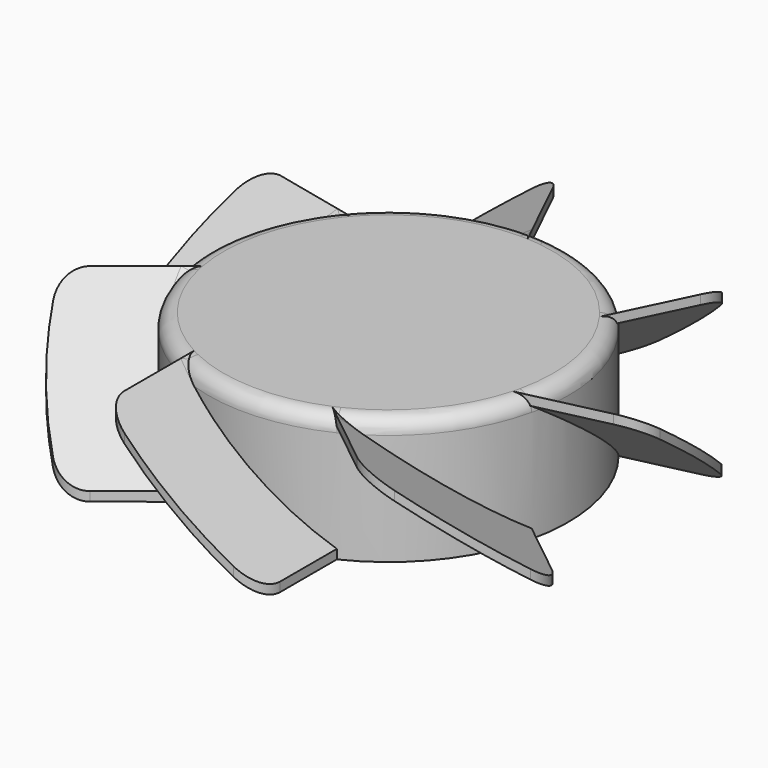
from build123d import *

# Parameters (mm, degrees)
F1_DEPTH       = 8.5
F3_DEPTH       = 10
F5_DEPTH       = 10
F7_DEPTH       = 10
F9_DEPTH       = 10
F11_DEPTH      = 10
F13_DEPTH      = 10
F15_DEPTH      = 10
F16_R          = 12.1
F17_DEPTH      = 8.5
F18_R          = 25
F18_R_2        = 18
F19_DEPTH      = 8.5
F20_R          = 2.5
F21_DEPTH      = 5
F22_T1_DEPTH   = 8.8499746994
F22_T3_DEPTH   = 8.8499746994
F23_T4_ANGLE   = 51.4285714286
F23_T9_ANGLE   = 51.4285714286
F23_T15_ANGLE  = 51.4285714286
F23_T21_ANGLE  = 51.4285714286
F23_T26_ANGLE  = 51.4285714286
F23_T32_ANGLE  = 51.4285714286
F23_T38_ANGLE  = 51.4285714286
F23_T43_ANGLE  = 51.4285714286
F23_T48_ANGLE  = 51.4285714286
F23_T53_ANGLE  = 51.4285714286
F23_T59_ANGLE  = 51.4285714286
F23_T65_ANGLE  = 51.4285714286
F23_T70_ANGLE  = 51.4285714286
F23_T75_ANGLE  = 51.4285714286
F23_T81_ANGLE  = 51.4285714286
F23_T87_ANGLE  = 51.4285714286
F23_T92_ANGLE  = 51.4285714286
F23_T97_ANGLE  = 51.4285714286
F23_T103_ANGLE = 51.4285714286
F23_T109_ANGLE = 51.4285714286
F23_T114_ANGLE = 51.4285714286
F23_T119_ANGLE = 51.4285714286
F23_T125_ANGLE = 51.4285714286
F23_T131_ANGLE = 51.4285714286
F23_T136_ANGLE = 51.4285714286
F23_T141_ANGLE = 51.4285714286
F23_T147_ANGLE = 51.4285714286
F23_T153_ANGLE = 51.4285714286


# Not quite as in the source:
# - a fillet or chamfer that OpenCascade refuses, or shapes differently, is made with other operations: its cross-section is extruded or revolved along the edge and cut away or added


with BuildPart() as f1:
    # F0 (on Top) → F1 (new body)
    with BuildSketch(Plane.XY):
        Polygon((9.4601609379, 7.5442266025), (0, 12.1), (-9.4601609379, 7.5442266025), (-11.7966277374, -2.6925033009), (-5.2499932433, -10.9017233016), (5.2499932433, -10.9017233016), (11.7966277374, -2.6925033009), align=None)
    extrude(amount=F1_DEPTH)

    # F2 (on face) → F3 (join)
    with BuildSketch(Plane(origin=(-10.6283943376, 2.4258616508, 0), x_dir=(-0.222520934, -0.9749279122, 0), z_dir=(-0.9749279122, 0.222520934, 0))):
        Polygon((5.2499932433, 0.6250002815), (-5.2499932433, 8.5), (-5.2499932433, 7.8749997185), (5.2499932433, 0), align=None)
    extrude(amount=F3_DEPTH)

    # F4 (on face) → F5 (join)
    with BuildSketch(Plane(origin=(-8.5233104904, -6.7971133012, 0), x_dir=(0.6234898019, -0.7818314825, 0), z_dir=(-0.7818314825, -0.6234898019, 0))):
        Polygon((5.2499932433, 0.6250002815), (-5.2499932433, 8.5), (-5.2499932433, 7.8749997185), (5.2499932433, 0), align=None)
    extrude(amount=F5_DEPTH)

    # F6 (on face) → F7 (join)
    with BuildSketch(Plane.XZ.offset(10.9017233016)):
        Polygon((5.2499932433, 0.6250002815), (-5.2499932433, 8.5), (-5.2499932433, 7.8749997185), (5.2499932433, 0), align=None)
    extrude(amount=F7_DEPTH)

    # F8 (on face) → F9 (join)
    with BuildSketch(Plane(origin=(8.5233104904, -6.7971133012, 0), x_dir=(0.6234898019, 0.7818314825, 0), z_dir=(0.7818314825, -0.6234898019, 0))):
        Polygon((5.2499932433, 0.6250002815), (-5.2499932433, 8.5), (-5.2499932433, 7.8749997185), (5.2499932433, 0), align=None)
    extrude(amount=F9_DEPTH)

    # F10 (on face) → F11 (join)
    with BuildSketch(Plane(origin=(10.6283943376, 2.4258616508, 0), x_dir=(-0.222520934, 0.9749279122, 0), z_dir=(0.9749279122, 0.222520934, 0))):
        Polygon((5.2499932433, 0.6250002815), (-5.2499932433, 8.5), (-5.2499932433, 7.8749997185), (5.2499932433, 0), align=None)
    extrude(amount=F11_DEPTH)

    # F12 (on face) → F13 (join)
    with BuildSketch(Plane(origin=(4.7300804689, 9.8221133012, 0), x_dir=(-0.9009688679, 0.4338837391, 0), z_dir=(0.4338837391, 0.9009688679, 0))):
        Polygon((5.2499932433, 0.6250002815), (-5.2499932433, 8.5), (-5.2499932433, 7.8749997185), (5.2499932433, 0), align=None)
    extrude(amount=F13_DEPTH)

    # F14 (on face) → F15 (join)
    with BuildSketch(Plane(origin=(-4.7300804689, 9.8221133012, 0), x_dir=(-0.9009688679, -0.4338837391, 0), z_dir=(-0.4338837391, 0.9009688679, 0))):
        Polygon((5.2499932433, 0.6250002815), (-5.2499932433, 8.5), (-5.2499932433, 7.8749997185), (5.2499932433, 0), align=None)
    extrude(amount=F15_DEPTH)

    # F16 (on Top) → F17 (join)
    with BuildSketch(Plane.XY):
        Circle(F16_R)
    extrude(amount=F17_DEPTH)

    # F18 (on face) → F19 (cut, through all)
    with BuildSketch(Plane.XY.offset(8.5)):
        Circle(F18_R)
        Circle(F18_R_2, mode=Mode.SUBTRACT)
    extrude(amount=-F19_DEPTH, mode=Mode.SUBTRACT)

    # F20 (on face) → F21 (cut)
    with BuildSketch(Plane(origin=(0, 0, 0), x_dir=(1, 0, 0), z_dir=(0, 0, -1))):
        Circle(F20_R)
    extrude(amount=-F21_DEPTH, mode=Mode.SUBTRACT)

    # F22: fillet of radius 2 on 14 edges, made by hand

    # F22_s2 → F22_t1 (cut)
    with BuildSketch(Plane.XY.offset(3.7625125095)):
        with BuildLine():
            ThreePointArc((-5.2499932433, -15.6664464356), (-4.8012021768, -16.9288848874), (-3.6562423987, -17.62475224))
            ThreePointArc((-3.6562423987, -17.62475224), (-4.4577741005, -17.4392732093), (-5.2499932433, -17.2173624852))
            Line((-5.2499932433, -17.2173624852), (-5.2499932433, -15.6664464356))
        make_face()
        with BuildLine():
            ThreePointArc((8.9752037947, -13.8724795843), (10.2420345741, -14.3087180997), (11.4999563232, -13.8474186968))
            ThreePointArc((11.4999563232, -13.8474186968), (10.8551961357, -14.3584371313), (10.1877587889, -14.8394599248))
            Line((10.1877587889, -14.8394599248), (8.9752037947, -13.8724795843))
        make_face()
        with BuildLine():
            ThreePointArc((16.4418893145, -1.6322526591), (17.5728103913, -0.9137947383), (17.9964533774, 0.357303561))
            ThreePointArc((17.9964533774, 0.357303561), (17.9939822761, -0.4654050347), (17.9539206607, -1.2871413712))
            Line((17.9539206607, -1.2871413712), (16.4418893145, -1.6322526591))
        make_face()
        with BuildLine():
            ThreePointArc((11.5274968271, 11.8370938103), (11.6709015639, 13.1692346991), (10.9412539777, 14.2929689497))
            ThreePointArc((10.9412539777, 14.2929689497), (11.5829327522, 13.7780865456), (12.2004140817, 13.2344208878))
            Line((12.2004140817, 13.2344208878), (11.5274968271, 11.8370938103))
        make_face()
        with BuildLine():
            ThreePointArc((-2.0673358892, 16.3928672079), (-3.0194341842, 17.3355618046), (-4.3529328281, 17.4657371958))
            ThreePointArc((-4.3529328281, 17.4657371958), (-3.5503013829, 17.6463979353), (-2.7402531439, 17.7901942853))
            Line((-2.7402531439, 17.7901942853), (-2.0673358892, 16.3928672079))
        make_face()
        with BuildLine():
            ThreePointArc((-14.105422515, 8.6044772443), (-15.4360744063, 8.4478572902), (-16.3692724307, 7.4864490974))
            ThreePointArc((-16.3692724307, 7.4864490974), (-16.0100861637, 8.2266117588), (-15.6174538612, 8.9495885321))
            Line((-15.6174538612, 8.9495885321), (-14.105422515, 8.6044772443))
        make_face()
        with BuildLine():
            ThreePointArc((-15.5218382888, -5.6632595836), (-16.2290357619, -6.8012560686), (-16.0592160207, -8.1302878671))
            ThreePointArc((-16.0592160207, -8.1302878671), (-16.413949517, -7.3879808643), (-16.734393283, -6.630239924))
            Line((-16.734393283, -6.630239924), (-15.5218382888, -5.6632595836))
        make_face()
    extrude(amount=F22_T1_DEPTH, mode=Mode.SUBTRACT)

    # F22_s4 → F22_t3 (cut)
    with BuildSketch(Plane.XY.offset(-4.1124872089)):
        with BuildLine():
            ThreePointArc((5.2499932433, -15.6664464356), (4.8012021768, -16.9288848874), (3.6562423987, -17.62475224))
            ThreePointArc((3.6562423987, -17.62475224), (4.4577741005, -17.4392732093), (5.2499932433, -17.2173624852))
            Line((5.2499932433, -17.2173624852), (5.2499932433, -15.6664464356))
        make_face()
        with BuildLine():
            ThreePointArc((15.5218382888, -5.6632595836), (16.2290357619, -6.8012560686), (16.0592160207, -8.1302878671))
            ThreePointArc((16.0592160207, -8.1302878671), (16.413949517, -7.3879808643), (16.734393283, -6.630239924))
            Line((16.734393283, -6.630239924), (15.5218382888, -5.6632595836))
        make_face()
        with BuildLine():
            ThreePointArc((14.105422515, 8.6044772443), (15.4360744063, 8.4478572902), (16.3692724307, 7.4864490974))
            ThreePointArc((16.3692724307, 7.4864490974), (16.0100861637, 8.2266117588), (15.6174538612, 8.9495885321))
            Line((15.6174538612, 8.9495885321), (14.105422515, 8.6044772443))
        make_face()
        with BuildLine():
            ThreePointArc((2.0673358892, 16.3928672079), (3.0194341842, 17.3355618046), (4.3529328281, 17.4657371958))
            ThreePointArc((4.3529328281, 17.4657371958), (3.5503013829, 17.6463979353), (2.7402531439, 17.7901942853))
            Line((2.7402531439, 17.7901942853), (2.0673358892, 16.3928672079))
        make_face()
        with BuildLine():
            ThreePointArc((-11.5274968271, 11.8370938103), (-11.6709015639, 13.1692346991), (-10.9412539777, 14.2929689497))
            ThreePointArc((-10.9412539777, 14.2929689497), (-11.5829327522, 13.7780865456), (-12.2004140817, 13.2344208878))
            Line((-12.2004140817, 13.2344208878), (-11.5274968271, 11.8370938103))
        make_face()
        with BuildLine():
            ThreePointArc((-16.4418893145, -1.6322526591), (-17.5728103913, -0.9137947383), (-17.9964533774, 0.357303561))
            ThreePointArc((-17.9964533774, 0.357303561), (-17.9939822761, -0.4654050347), (-17.9539206607, -1.2871413712))
            Line((-17.9539206607, -1.2871413712), (-16.4418893145, -1.6322526591))
        make_face()
        with BuildLine():
            ThreePointArc((-8.9752037947, -13.8724795843), (-10.2420345741, -14.3087180997), (-11.4999563232, -13.8474186968))
            ThreePointArc((-11.4999563232, -13.8474186968), (-10.8551961357, -14.3584371313), (-10.1877587889, -14.8394599248))
            Line((-10.1877587889, -14.8394599248), (-8.9752037947, -13.8724795843))
        make_face()
    extrude(amount=F22_T3_DEPTH, mode=Mode.SUBTRACT)

    # F23: fillet of radius 1 on 7 edges, made by hand


with BuildPart() as f23_tool2:
    # F23_s3 → F23_t4 (revolve)
    with BuildSketch(Plane(origin=(0, 0, 0), x_dir=(0, 0, 1), z_dir=(-0.9009688679, -0.4338837391, 0))):
        with BuildLine():
            ThreePointArc((7.5, -12.1), (8.2071067812, -11.8071067812), (8.5, -11.1))
            Line((8.5, -11.1), (8.5, -12.1))
            Line((8.5, -12.1), (7.5, -12.1))
        make_face()
    revolve(axis=Axis((0, 0, 8.5), (0, 0, 1)), revolution_arc=F23_T4_ANGLE)

    split(bisect_by=Plane(origin=(1.1783960962, 1.4776619667, 2.5199976397), x_dir=(0.7818314825, -0.6234898019, 0), z_dir=(-0.3740941807, -0.4690992651, -0.7999996396)), keep=Keep.TOP)


with BuildPart() as f1_1:
    add(f1.part)

    # F23_t1: cut F23_tool2
    add(f23_tool2.part, mode=Mode.SUBTRACT)


with BuildPart() as f23_tool7:
    # F23_s8 → F23_t9 (revolve)
    with BuildSketch(Plane(origin=(0, 0, 0), x_dir=(0, 0, 1), z_dir=(-0.9009688679, -0.4338837391, 0))):
        with BuildLine():
            ThreePointArc((7.5, -12.1), (8.2071067812, -11.8071067812), (8.5, -11.1))
            Line((8.5, -11.1), (8.5, -12.1))
            Line((8.5, -12.1), (7.5, -12.1))
        make_face()
    revolve(axis=Axis((0, 0, 8.5), (0, 0, 1)), revolution_arc=F23_T9_ANGLE)

    split(bisect_by=Plane(origin=(1.3654431866, 1.7122115993, 2.9199974595), x_dir=(-0.7818314825, 0.6234898019, 0), z_dir=(0.3740941807, 0.4690992651, 0.7999996396)), keep=Keep.TOP)

    split(bisect_by=Plane(origin=(1.1682333998, -5.1183649517, 0), x_dir=(0, 0, 1), z_dir=(0.222520934, -0.9749279122, 0)), keep=Keep.TOP)


with BuildPart() as f1_2:
    add(f1_1.part)

    # F23_t6: cut F23_tool7
    add(f23_tool7.part, mode=Mode.SUBTRACT)


with BuildPart() as f23_tool13:
    # F23_s14 → F23_t15 (revolve)
    with BuildSketch(Plane(origin=(0, 0, 0), x_dir=(0, 0, 1), z_dir=(-0.9009688679, -0.4338837391, 0))):
        with BuildLine():
            ThreePointArc((7.5, -12.1), (8.2071067812, -11.8071067812), (8.5, -11.1))
            Line((8.5, -11.1), (8.5, -12.1))
            Line((8.5, -12.1), (7.5, -12.1))
        make_face()
    revolve(axis=Axis((0, 0, 8.5), (0, 0, 1)), revolution_arc=F23_T15_ANGLE)

    split(bisect_by=Plane(origin=(-0.4205646975, 1.8426143337, 2.5199976397), x_dir=(0.9749279122, 0.222520934, 0), z_dir=(0.1335126673, -0.5849572157, -0.7999996396)), keep=Keep.TOP)

    split(bisect_by=Plane(origin=(1.1682333998, -5.1183649517, 0), x_dir=(0, 0, 1), z_dir=(-0.222520934, 0.9749279122, 0)), keep=Keep.TOP)


with BuildPart() as f1_3:
    add(f1_2.part)

    # F23_t12: cut F23_tool13
    add(f23_tool13.part, mode=Mode.SUBTRACT)


with BuildPart() as f23_tool19:
    # F23_s20 → F23_t21 (revolve)
    with BuildSketch(Plane(origin=(0, 0, 0), x_dir=(0, 0, 1), z_dir=(-0.9009688679, -0.4338837391, 0))):
        with BuildLine():
            ThreePointArc((7.5, -12.1), (8.2071067812, -11.8071067812), (8.5, -11.1))
            Line((8.5, -11.1), (8.5, -12.1))
            Line((8.5, -12.1), (7.5, -12.1))
        make_face()
    revolve(axis=Axis((0, 0, 8.5), (0, 0, 1)), revolution_arc=F23_T21_ANGLE)

    split(bisect_by=Plane(origin=(-0.4873210311, 2.1350929416, 2.9199974595), x_dir=(-0.9749279122, -0.222520934, 0), z_dir=(-0.1335126673, 0.5849572157, 0.7999996396)), keep=Keep.TOP)


with BuildPart() as f1_4:
    add(f1_3.part)

    # F23_t18: cut F23_tool19
    add(f23_tool19.part, mode=Mode.SUBTRACT)


with BuildPart() as f23_tool24:
    # F23_s25 → F23_t26 (revolve)
    with BuildSketch(Plane(origin=(0, 0, 0), x_dir=(0, 0, 1), z_dir=(-0.6234898019, 0.7818314825, 0))):
        with BuildLine():
            ThreePointArc((7.5, 12.1), (8.2071067812, 11.8071067812), (8.5, 11.1))
            Line((8.5, 11.1), (8.5, 12.1))
            Line((8.5, 12.1), (7.5, 12.1))
        make_face()
    revolve(axis=Axis((0, 0, 8.5), (0, 0, -1)), revolution_arc=F23_T26_ANGLE)

    split(bisect_by=Plane(origin=(-0.4873210311, 2.1350929416, 2.9199974595), x_dir=(-0.9749279122, -0.222520934, 0), z_dir=(-0.1335126673, 0.5849572157, 0.7999996396)), keep=Keep.TOP)

    split(bisect_by=Plane(origin=(-1.702831696, 0.8200405249, 2.5199976397), x_dir=(0.4338837391, 0.9009688679, 0), z_dir=(0.5405817536, -0.2603304519, -0.7999996396)), keep=Keep.TOP)


with BuildPart() as f1_5:
    add(f1_4.part)

    # F23_t23: cut F23_tool24
    add(f23_tool24.part, mode=Mode.SUBTRACT)


with BuildPart() as f23_tool30:
    # F23_s31 → F23_t32 (revolve)
    with BuildSketch(Plane(origin=(0, 0, 0), x_dir=(0, 0, 1), z_dir=(-0.6234898019, 0.7818314825, 0))):
        with BuildLine():
            ThreePointArc((7.5, 12.1), (8.2071067812, 11.8071067812), (8.5, 11.1))
            Line((8.5, 11.1), (8.5, 12.1))
            Line((8.5, 12.1), (7.5, 12.1))
        make_face()
    revolve(axis=Axis((0, 0, 8.5), (0, 0, -1)), revolution_arc=F23_T32_ANGLE)

    split(bisect_by=Plane(origin=(4.7300804689, -2.2778866988, 0), x_dir=(0, 0, 1), z_dir=(0.9009688679, -0.4338837391, 0)), keep=Keep.TOP)

    split(bisect_by=Plane(origin=(-1.702831696, 0.8200405249, 2.5199976397), x_dir=(-0.4338837391, -0.9009688679, 0), z_dir=(-0.5405817536, 0.2603304519, 0.7999996396)), keep=Keep.TOP)


with BuildPart() as f1_6:
    add(f1_5.part)

    # F23_t29: cut F23_tool30
    add(f23_tool30.part, mode=Mode.SUBTRACT)


with BuildPart() as f23_tool36:
    # F23_s37 → F23_t38 (revolve)
    with BuildSketch(Plane(origin=(0, 0, 0), x_dir=(0, 0, 1), z_dir=(-0.6234898019, 0.7818314825, 0))):
        with BuildLine():
            ThreePointArc((7.5, 12.1), (8.2071067812, 11.8071067812), (8.5, 11.1))
            Line((8.5, 11.1), (8.5, 12.1))
            Line((8.5, 12.1), (7.5, 12.1))
        make_face()
    revolve(axis=Axis((0, 0, 8.5), (0, 0, -1)), revolution_arc=F23_T38_ANGLE)

    split(bisect_by=Plane(origin=(-0.4205646975, 1.8426143337, 2.5199976397), x_dir=(0.9749279122, 0.222520934, 0), z_dir=(0.1335126673, -0.5849572157, -0.7999996396)), keep=Keep.TOP)


with BuildPart() as f1_7:
    add(f1_6.part)

    # F23_t35: cut F23_tool36
    add(f23_tool36.part, mode=Mode.SUBTRACT)


with BuildPart() as f23_tool41:
    # F23_s42 → F23_t43 (revolve)
    with BuildSketch(Plane(origin=(0, 0, 0), x_dir=(0, 0, 1), z_dir=(-0.6234898019, 0.7818314825, 0))):
        with BuildLine():
            ThreePointArc((7.5, 12.1), (8.2071067812, 11.8071067812), (8.5, 11.1))
            Line((8.5, 11.1), (8.5, 12.1))
            Line((8.5, 12.1), (7.5, 12.1))
        make_face()
    revolve(axis=Axis((0, 0, 8.5), (0, 0, -1)), revolution_arc=F23_T43_ANGLE)

    split(bisect_by=Plane(origin=(-1.9731225729, 0.9502057509, 2.9199974595), x_dir=(-0.4338837391, -0.9009688679, 0), z_dir=(-0.5405817536, 0.2603304519, 0.7999996396)), keep=Keep.TOP)


with BuildPart() as f1_8:
    add(f1_7.part)

    # F23_t40: cut F23_tool41
    add(f23_tool41.part, mode=Mode.SUBTRACT)


with BuildPart() as f23_tool46:
    # F23_s47 → F23_t48 (revolve)
    with BuildSketch(Plane(origin=(0, 0, 0), x_dir=(0, 0, 1), z_dir=(0.6234898019, -0.7818314825, 0))):
        with BuildLine():
            ThreePointArc((7.5, -12.1), (8.2071067812, -11.8071067812), (8.5, -11.1))
            Line((8.5, -11.1), (8.5, -12.1))
            Line((8.5, -12.1), (7.5, -12.1))
        make_face()
    revolve(axis=Axis((0, 0, 8.5), (0, 0, 1)), revolution_arc=F23_T48_ANGLE)

    split(bisect_by=Plane(origin=(-1.702831696, 0.8200405249, 2.5199976397), x_dir=(0.4338837391, 0.9009688679, 0), z_dir=(0.5405817536, -0.2603304519, -0.7999996396)), keep=Keep.TOP)


with BuildPart() as f1_9:
    add(f1_8.part)

    # F23_t45: cut F23_tool46
    add(f23_tool46.part, mode=Mode.SUBTRACT)


with BuildPart() as f23_tool51:
    # F23_s52 → F23_t53 (revolve)
    with BuildSketch(Plane(origin=(0, 0, 0), x_dir=(0, 0, 1), z_dir=(0.6234898019, -0.7818314825, 0))):
        with BuildLine():
            ThreePointArc((7.5, -12.1), (8.2071067812, -11.8071067812), (8.5, -11.1))
            Line((8.5, -11.1), (8.5, -12.1))
            Line((8.5, -12.1), (7.5, -12.1))
        make_face()
    revolve(axis=Axis((0, 0, 8.5), (0, 0, 1)), revolution_arc=F23_T53_ANGLE)

    split(bisect_by=Plane(origin=(-1.9731225729, 0.9502057509, 2.9199974595), x_dir=(-0.4338837391, -0.9009688679, 0), z_dir=(-0.5405817536, 0.2603304519, 0.7999996396)), keep=Keep.TOP)

    split(bisect_by=Plane(origin=(-1.702831696, -0.8200405249, 2.5199976397), x_dir=(-0.4338837391, 0.9009688679, 0), z_dir=(0.5405817536, 0.2603304519, -0.7999996396)), keep=Keep.TOP)


with BuildPart() as f1_10:
    add(f1_9.part)

    # F23_t50: cut F23_tool51
    add(f23_tool51.part, mode=Mode.SUBTRACT)


with BuildPart() as f23_tool57:
    # F23_s58 → F23_t59 (revolve)
    with BuildSketch(Plane(origin=(0, 0, 0), x_dir=(0, 0, 1), z_dir=(0.6234898019, -0.7818314825, 0))):
        with BuildLine():
            ThreePointArc((7.5, -12.1), (8.2071067812, -11.8071067812), (8.5, -11.1))
            Line((8.5, -11.1), (8.5, -12.1))
            Line((8.5, -12.1), (7.5, -12.1))
        make_face()
    revolve(axis=Axis((0, 0, 8.5), (0, 0, 1)), revolution_arc=F23_T59_ANGLE)

    split(bisect_by=Plane(origin=(4.7300804689, 2.2778866988, 0), x_dir=(0, 0, 1), z_dir=(0.9009688679, 0.4338837391, 0)), keep=Keep.TOP)

    split(bisect_by=Plane(origin=(-1.702831696, -0.8200405249, 2.5199976397), x_dir=(0.4338837391, -0.9009688679, 0), z_dir=(-0.5405817536, -0.2603304519, 0.7999996396)), keep=Keep.TOP)


with BuildPart() as f1_11:
    add(f1_10.part)

    # F23_t56: cut F23_tool57
    add(f23_tool57.part, mode=Mode.SUBTRACT)


with BuildPart() as f23_tool63:
    # F23_s64 → F23_t65 (revolve)
    with BuildSketch(Plane(origin=(0, 0, 0), x_dir=(0, 0, 1), z_dir=(0.6234898019, -0.7818314825, 0))):
        with BuildLine():
            ThreePointArc((7.5, -12.1), (8.2071067812, -11.8071067812), (8.5, -11.1))
            Line((8.5, -11.1), (8.5, -12.1))
            Line((8.5, -12.1), (7.5, -12.1))
        make_face()
    revolve(axis=Axis((0, 0, 8.5), (0, 0, 1)), revolution_arc=F23_T65_ANGLE)

    split(bisect_by=Plane(origin=(-1.9731225729, -0.9502057509, 2.9199974595), x_dir=(0.4338837391, -0.9009688679, 0), z_dir=(-0.5405817536, -0.2603304519, 0.7999996396)), keep=Keep.TOP)


with BuildPart() as f1_12:
    add(f1_11.part)

    # F23_t62: cut F23_tool63
    add(f23_tool63.part, mode=Mode.SUBTRACT)


with BuildPart() as f23_tool68:
    # F23_s69 → F23_t70 (revolve)
    with BuildSketch(Plane.YZ):
        with BuildLine():
            ThreePointArc((12.1, 7.5), (11.8071067812, 8.2071067812), (11.1, 8.5))
            Line((11.1, 8.5), (12.1, 8.5))
            Line((12.1, 8.5), (12.1, 7.5))
        make_face()
    revolve(axis=Axis((0, 0, 8.5), (0, 0, 1)), revolution_arc=F23_T70_ANGLE)

    split(bisect_by=Plane(origin=(-1.702831696, -0.8200405249, 2.5199976397), x_dir=(-0.4338837391, 0.9009688679, 0), z_dir=(0.5405817536, 0.2603304519, -0.7999996396)), keep=Keep.TOP)


with BuildPart() as f1_13:
    add(f1_12.part)

    # F23_t67: cut F23_tool68
    add(f23_tool68.part, mode=Mode.SUBTRACT)


with BuildPart() as f23_tool73:
    # F23_s74 → F23_t75 (revolve)
    with BuildSketch(Plane.YZ):
        with BuildLine():
            ThreePointArc((12.1, 7.5), (11.8071067812, 8.2071067812), (11.1, 8.5))
            Line((11.1, 8.5), (12.1, 8.5))
            Line((12.1, 8.5), (12.1, 7.5))
        make_face()
    revolve(axis=Axis((0, 0, 8.5), (0, 0, 1)), revolution_arc=F23_T75_ANGLE)

    split(bisect_by=Plane(origin=(-1.9731225729, -0.9502057509, 2.9199974595), x_dir=(0.4338837391, -0.9009688679, 0), z_dir=(-0.5405817536, -0.2603304519, 0.7999996396)), keep=Keep.TOP)

    split(bisect_by=Plane(origin=(-0.4205646975, -1.8426143337, 2.5199976397), x_dir=(-0.9749279122, 0.222520934, 0), z_dir=(0.1335126673, 0.5849572157, -0.7999996396)), keep=Keep.TOP)


with BuildPart() as f1_14:
    add(f1_13.part)

    # F23_t72: cut F23_tool73
    add(f23_tool73.part, mode=Mode.SUBTRACT)


with BuildPart() as f23_tool79:
    # F23_s80 → F23_t81 (revolve)
    with BuildSketch(Plane.YZ):
        with BuildLine():
            ThreePointArc((12.1, 7.5), (11.8071067812, 8.2071067812), (11.1, 8.5))
            Line((11.1, 8.5), (12.1, 8.5))
            Line((12.1, 8.5), (12.1, 7.5))
        make_face()
    revolve(axis=Axis((0, 0, 8.5), (0, 0, 1)), revolution_arc=F23_T81_ANGLE)

    split(bisect_by=Plane(origin=(1.1682333998, 5.1183649517, 0), x_dir=(0, 0, 1), z_dir=(0.222520934, 0.9749279122, 0)), keep=Keep.TOP)

    split(bisect_by=Plane(origin=(-0.4205646975, -1.8426143337, 2.5199976397), x_dir=(0.9749279122, -0.222520934, 0), z_dir=(-0.1335126673, -0.5849572157, 0.7999996396)), keep=Keep.TOP)


with BuildPart() as f1_15:
    add(f1_14.part)

    # F23_t78: cut F23_tool79
    add(f23_tool79.part, mode=Mode.SUBTRACT)


with BuildPart() as f23_tool85:
    # F23_s86 → F23_t87 (revolve)
    with BuildSketch(Plane.YZ):
        with BuildLine():
            ThreePointArc((12.1, 7.5), (11.8071067812, 8.2071067812), (11.1, 8.5))
            Line((11.1, 8.5), (12.1, 8.5))
            Line((12.1, 8.5), (12.1, 7.5))
        make_face()
    revolve(axis=Axis((0, 0, 8.5), (0, 0, 1)), revolution_arc=F23_T87_ANGLE)

    split(bisect_by=Plane(origin=(-0.4873210311, -2.1350929416, 2.9199974595), x_dir=(0.9749279122, -0.222520934, 0), z_dir=(-0.1335126673, -0.5849572157, 0.7999996396)), keep=Keep.TOP)


with BuildPart() as f1_16:
    add(f1_15.part)

    # F23_t84: cut F23_tool85
    add(f23_tool85.part, mode=Mode.SUBTRACT)


with BuildPart() as f23_tool90:
    # F23_s91 → F23_t92 (revolve)
    with BuildSketch(Plane(origin=(0, 0, 0), x_dir=(0, 0, 1), z_dir=(0.6234898019, 0.7818314825, 0))):
        with BuildLine():
            ThreePointArc((7.5, -12.1), (8.2071067812, -11.8071067812), (8.5, -11.1))
            Line((8.5, -11.1), (8.5, -12.1))
            Line((8.5, -12.1), (7.5, -12.1))
        make_face()
    revolve(axis=Axis((0, 0, 8.5), (0, 0, 1)), revolution_arc=F23_T92_ANGLE)

    split(bisect_by=Plane(origin=(-0.4205646975, -1.8426143337, 2.5199976397), x_dir=(-0.9749279122, 0.222520934, 0), z_dir=(0.1335126673, 0.5849572157, -0.7999996396)), keep=Keep.TOP)


with BuildPart() as f1_17:
    add(f1_16.part)

    # F23_t89: cut F23_tool90
    add(f23_tool90.part, mode=Mode.SUBTRACT)


with BuildPart() as f23_tool95:
    # F23_s96 → F23_t97 (revolve)
    with BuildSketch(Plane(origin=(0, 0, 0), x_dir=(0, 0, 1), z_dir=(0.6234898019, 0.7818314825, 0))):
        with BuildLine():
            ThreePointArc((7.5, -12.1), (8.2071067812, -11.8071067812), (8.5, -11.1))
            Line((8.5, -11.1), (8.5, -12.1))
            Line((8.5, -12.1), (7.5, -12.1))
        make_face()
    revolve(axis=Axis((0, 0, 8.5), (0, 0, 1)), revolution_arc=F23_T97_ANGLE)

    split(bisect_by=Plane(origin=(-0.4873210311, -2.1350929416, 2.9199974595), x_dir=(0.9749279122, -0.222520934, 0), z_dir=(-0.1335126673, -0.5849572157, 0.7999996396)), keep=Keep.TOP)

    split(bisect_by=Plane(origin=(-3.273317247, 4.1046100004, 0), x_dir=(0, 0, 1), z_dir=(-0.6234898019, 0.7818314825, 0)), keep=Keep.TOP)


with BuildPart() as f1_18:
    add(f1_17.part)

    # F23_t94: cut F23_tool95
    add(f23_tool95.part, mode=Mode.SUBTRACT)


with BuildPart() as f23_tool101:
    # F23_s102 → F23_t103 (revolve)
    with BuildSketch(Plane(origin=(0, 0, 0), x_dir=(0, 0, 1), z_dir=(0.6234898019, 0.7818314825, 0))):
        with BuildLine():
            ThreePointArc((7.5, -12.1), (8.2071067812, -11.8071067812), (8.5, -11.1))
            Line((8.5, -11.1), (8.5, -12.1))
            Line((8.5, -12.1), (7.5, -12.1))
        make_face()
    revolve(axis=Axis((0, 0, 8.5), (0, 0, 1)), revolution_arc=F23_T103_ANGLE)

    split(bisect_by=Plane(origin=(1.1783960962, -1.4776619667, 2.5199976397), x_dir=(-0.7818314825, -0.6234898019, 0), z_dir=(-0.3740941807, 0.4690992651, -0.7999996396)), keep=Keep.TOP)

    split(bisect_by=Plane(origin=(-3.273317247, 4.1046100004, 0), x_dir=(0, 0, 1), z_dir=(0.6234898019, -0.7818314825, 0)), keep=Keep.TOP)


with BuildPart() as f1_19:
    add(f1_18.part)

    # F23_t100: cut F23_tool101
    add(f23_tool101.part, mode=Mode.SUBTRACT)


with BuildPart() as f23_tool107:
    # F23_s108 → F23_t109 (revolve)
    with BuildSketch(Plane(origin=(0, 0, 0), x_dir=(0, 0, 1), z_dir=(0.6234898019, 0.7818314825, 0))):
        with BuildLine():
            ThreePointArc((7.5, -12.1), (8.2071067812, -11.8071067812), (8.5, -11.1))
            Line((8.5, -11.1), (8.5, -12.1))
            Line((8.5, -12.1), (7.5, -12.1))
        make_face()
    revolve(axis=Axis((0, 0, 8.5), (0, 0, 1)), revolution_arc=F23_T109_ANGLE)

    split(bisect_by=Plane(origin=(1.3654431866, -1.7122115993, 2.9199974595), x_dir=(0.7818314825, 0.6234898019, 0), z_dir=(0.3740941807, -0.4690992651, 0.7999996396)), keep=Keep.TOP)


with BuildPart() as f1_20:
    add(f1_19.part)

    # F23_t106: cut F23_tool107
    add(f23_tool107.part, mode=Mode.SUBTRACT)


with BuildPart() as f23_tool112:
    # F23_s113 → F23_t114 (revolve)
    with BuildSketch(Plane(origin=(0, 0, 0), x_dir=(0, 0, 1), z_dir=(-0.222520934, 0.9749279122, 0))):
        with BuildLine():
            ThreePointArc((7.5, -12.1), (8.2071067812, -11.8071067812), (8.5, -11.1))
            Line((8.5, -11.1), (8.5, -12.1))
            Line((8.5, -12.1), (7.5, -12.1))
        make_face()
    revolve(axis=Axis((0, 0, 8.5), (0, 0, 1)), revolution_arc=F23_T114_ANGLE)

    split(bisect_by=Plane(origin=(1.1783960962, -1.4776619667, 2.5199976397), x_dir=(-0.7818314825, -0.6234898019, 0), z_dir=(-0.3740941807, 0.4690992651, -0.7999996396)), keep=Keep.TOP)


with BuildPart() as f1_21:
    add(f1_20.part)

    # F23_t111: cut F23_tool112
    add(f23_tool112.part, mode=Mode.SUBTRACT)


with BuildPart() as f23_tool117:
    # F23_s118 → F23_t119 (revolve)
    with BuildSketch(Plane(origin=(0, 0, 0), x_dir=(0, 0, 1), z_dir=(-0.222520934, 0.9749279122, 0))):
        with BuildLine():
            ThreePointArc((7.5, -12.1), (8.2071067812, -11.8071067812), (8.5, -11.1))
            Line((8.5, -11.1), (8.5, -12.1))
            Line((8.5, -12.1), (7.5, -12.1))
        make_face()
    revolve(axis=Axis((0, 0, 8.5), (0, 0, 1)), revolution_arc=F23_T119_ANGLE)

    split(bisect_by=Plane(origin=(1.3654431866, -1.7122115993, 2.9199974595), x_dir=(0.7818314825, 0.6234898019, 0), z_dir=(0.3740941807, -0.4690992651, 0.7999996396)), keep=Keep.TOP)

    split(bisect_by=Plane.YZ.offset(-5.2499932433), keep=Keep.BOTTOM)


with BuildPart() as f1_22:
    add(f1_21.part)

    # F23_t116: cut F23_tool117
    add(f23_tool117.part, mode=Mode.SUBTRACT)


with BuildPart() as f23_tool123:
    # F23_s124 → F23_t125 (revolve)
    with BuildSketch(Plane(origin=(0, 0, 0), x_dir=(0, 0, 1), z_dir=(-0.222520934, 0.9749279122, 0))):
        with BuildLine():
            ThreePointArc((7.5, -12.1), (8.2071067812, -11.8071067812), (8.5, -11.1))
            Line((8.5, -11.1), (8.5, -12.1))
            Line((8.5, -12.1), (7.5, -12.1))
        make_face()
    revolve(axis=Axis((0, 0, 8.5), (0, 0, 1)), revolution_arc=F23_T125_ANGLE)

    split(bisect_by=Plane(origin=(1.8900005946, 0, 2.5199976397), x_dir=(0, 1, 0), z_dir=(-0.6000004805, 0, -0.7999996396)), keep=Keep.TOP)

    split(bisect_by=Plane.YZ.offset(-5.2499932433), keep=Keep.TOP)


with BuildPart() as f1_23:
    add(f1_22.part)

    # F23_t122: cut F23_tool123
    add(f23_tool123.part, mode=Mode.SUBTRACT)


with BuildPart() as f23_tool129:
    # F23_s130 → F23_t131 (revolve)
    with BuildSketch(Plane(origin=(0, 0, 0), x_dir=(0, 0, 1), z_dir=(-0.222520934, 0.9749279122, 0))):
        with BuildLine():
            ThreePointArc((7.5, -12.1), (8.2071067812, -11.8071067812), (8.5, -11.1))
            Line((8.5, -11.1), (8.5, -12.1))
            Line((8.5, -12.1), (7.5, -12.1))
        make_face()
    revolve(axis=Axis((0, 0, 8.5), (0, 0, 1)), revolution_arc=F23_T131_ANGLE)

    split(bisect_by=Plane(origin=(2.1900008348, 0, 2.9199974595), x_dir=(0, 1, 0), z_dir=(0.6000004805, 0, 0.7999996396)), keep=Keep.TOP)


with BuildPart() as f1_24:
    add(f1_23.part)

    # F23_t128: cut F23_tool129
    add(f23_tool129.part, mode=Mode.SUBTRACT)


with BuildPart() as f23_tool134:
    # F23_s135 → F23_t136 (revolve)
    with BuildSketch(Plane(origin=(0, 0, 0), x_dir=(0, 0, 1), z_dir=(-0.9009688679, 0.4338837391, 0))):
        with BuildLine():
            ThreePointArc((7.5, -12.1), (8.2071067812, -11.8071067812), (8.5, -11.1))
            Line((8.5, -11.1), (8.5, -12.1))
            Line((8.5, -12.1), (7.5, -12.1))
        make_face()
    revolve(axis=Axis((0, 0, 8.5), (0, 0, 1)), revolution_arc=F23_T136_ANGLE)

    split(bisect_by=Plane(origin=(1.8900005946, 0, 2.5199976397), x_dir=(0, 1, 0), z_dir=(-0.6000004805, 0, -0.7999996396)), keep=Keep.TOP)


with BuildPart() as f1_25:
    add(f1_24.part)

    # F23_t133: cut F23_tool134
    add(f23_tool134.part, mode=Mode.SUBTRACT)


with BuildPart() as f23_tool139:
    # F23_s140 → F23_t141 (revolve)
    with BuildSketch(Plane(origin=(0, 0, 0), x_dir=(0, 0, 1), z_dir=(-0.9009688679, 0.4338837391, 0))):
        with BuildLine():
            ThreePointArc((7.5, -12.1), (8.2071067812, -11.8071067812), (8.5, -11.1))
            Line((8.5, -11.1), (8.5, -12.1))
            Line((8.5, -12.1), (7.5, -12.1))
        make_face()
    revolve(axis=Axis((0, 0, 8.5), (0, 0, 1)), revolution_arc=F23_T141_ANGLE)

    split(bisect_by=Plane(origin=(2.1900008348, 0, 2.9199974595), x_dir=(0, 1, 0), z_dir=(0.6000004805, 0, 0.7999996396)), keep=Keep.TOP)

    split(bisect_by=Plane(origin=(-3.273317247, -4.1046100004, 0), x_dir=(0, 0, 1), z_dir=(-0.6234898019, -0.7818314825, 0)), keep=Keep.TOP)


with BuildPart() as f1_26:
    add(f1_25.part)

    # F23_t138: cut F23_tool139
    add(f23_tool139.part, mode=Mode.SUBTRACT)


with BuildPart() as f23_tool145:
    # F23_s146 → F23_t147 (revolve)
    with BuildSketch(Plane(origin=(0, 0, 0), x_dir=(0, 0, 1), z_dir=(-0.9009688679, 0.4338837391, 0))):
        with BuildLine():
            ThreePointArc((7.5, -12.1), (8.2071067812, -11.8071067812), (8.5, -11.1))
            Line((8.5, -11.1), (8.5, -12.1))
            Line((8.5, -12.1), (7.5, -12.1))
        make_face()
    revolve(axis=Axis((0, 0, 8.5), (0, 0, 1)), revolution_arc=F23_T147_ANGLE)

    split(bisect_by=Plane(origin=(1.1783960962, 1.4776619667, 2.5199976397), x_dir=(0.7818314825, -0.6234898019, 0), z_dir=(-0.3740941807, -0.4690992651, -0.7999996396)), keep=Keep.TOP)

    split(bisect_by=Plane(origin=(-3.273317247, -4.1046100004, 0), x_dir=(0, 0, 1), z_dir=(0.6234898019, 0.7818314825, 0)), keep=Keep.TOP)


with BuildPart() as f1_27:
    add(f1_26.part)

    # F23_t144: cut F23_tool145
    add(f23_tool145.part, mode=Mode.SUBTRACT)


with BuildPart() as f23_tool151:
    # F23_s152 → F23_t153 (revolve)
    with BuildSketch(Plane(origin=(0, 0, 0), x_dir=(0, 0, 1), z_dir=(-0.9009688679, 0.4338837391, 0))):
        with BuildLine():
            ThreePointArc((7.5, -12.1), (8.2071067812, -11.8071067812), (8.5, -11.1))
            Line((8.5, -11.1), (8.5, -12.1))
            Line((8.5, -12.1), (7.5, -12.1))
        make_face()
    revolve(axis=Axis((0, 0, 8.5), (0, 0, 1)), revolution_arc=F23_T153_ANGLE)

    split(bisect_by=Plane(origin=(1.3654431866, 1.7122115993, 2.9199974595), x_dir=(-0.7818314825, 0.6234898019, 0), z_dir=(0.3740941807, 0.4690992651, 0.7999996396)), keep=Keep.TOP)


with BuildPart() as f1_28:
    add(f1_27.part)

    # F23_t150: cut F23_tool151
    add(f23_tool151.part, mode=Mode.SUBTRACT)


solid = f1_28.part
